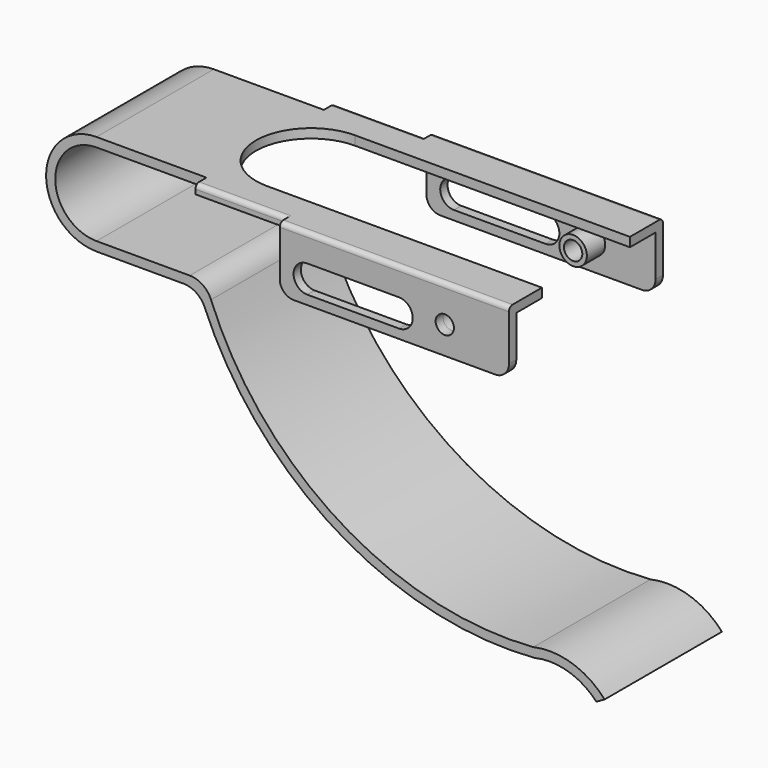
from build123d import *

# Parameters (mm, degrees)
F1_DEPTH  = 16
F2_W      = 70
F2_H      = 3
F3_DEPTH  = 2
F4_W      = 50
F4_H      = 14
F5_DEPTH  = 2
F6_R      = 1
F9_DEPTH  = 2
F11_DEPTH = 42.001
F13_D     = 4
F14_R     = 3
F14_R_2   = 2
F15_DEPTH = 5
F16_R     = 3


# Not quite as in the source:
# - a pattern or mirror of a feature is missing from the dataset's text; its kind, count and spacing are read off the source's solid


with BuildPart() as f1:
    # F0 (on Front) → F1 (new body)
    with BuildSketch(Plane.XZ):
        with BuildLine():
            ThreePointArc((0, -9), (-9, 0), (0, 9))
            Line((0, 9), (94, 9))
            Line((94, 9), (94, 11))
            Line((94, 11), (0, 11))
            ThreePointArc((0, 11), (-11, 0), (0, -11))
            Line((0, -11), (19, -11))
            ThreePointArc((19, -11), (21.7681124643, -11.8361612201), (23.6103896104, -14.064978646))
            ThreePointArc((23.6103896104, -14.064978646), (52.5045279084, -47.666837229), (95.6038093767, -57.9822657286))
            ThreePointArc((95.6038093767, -57.9822657286), (102.8775016632, -58.177663117), (109.0707194958, -61.9971961375))
            Line((109.0707194958, -61.9971961375), (110.8678187413, -61))
            ThreePointArc((110.8678187413, -61), (103.7692922231, -56.3602117831), (95.2965735981, -56))
            ThreePointArc((95.2965735981, -56), (52.955209083, -45.5949761441), (24.9861322889, -12.1467114099))
            ThreePointArc((24.9861322889, -12.1467114099), (23.1470623984, -9.8607704249), (20.3422845953, -9))
            Line((20.3422845953, -9), (0, -9))
        make_face()
    extrude(amount=F1_DEPTH)

    # F2 (on face) → F3 (join)
    with BuildSketch(Plane.XY.offset(11)):
        with Locations((59, -17.5)):
            Rectangle(F2_W, F2_H)
    extrude(amount=-F3_DEPTH)

    # F4 (on face) → F5 (join)
    with BuildSketch(Plane.XZ.offset(19)):
        with Locations((69, 4)):
            Rectangle(F4_W, F4_H)
    extrude(amount=F5_DEPTH)

    # F6
    f6_edges = [f1.edges().sort_by_distance(p)[0] for p in [
        (69, -21, 11),
        (34, -19, 11),
    ]]
    fillet(f6_edges, radius=F6_R)

    # F7: F1 across plane


with BuildPart() as f1_1:
    add(f1.part)
    add(f1.part.mirror(Plane.XZ))

    # F8 (on face) → F9 (cut)
    with BuildSketch(Plane.XY.offset(11)):
        with BuildLine():
            Line((94, 12), (34, 12))
            ThreePointArc((34, 12), (22, 0), (34, -12))
            Line((34, -12), (94, -12))
            Line((94, -12), (94, 12))
        make_face()
    extrude(amount=-F9_DEPTH, mode=Mode.SUBTRACT)

    # F10 (on face) → F11 (cut, through all)
    with BuildSketch(Plane.XZ.offset(21)):
        with BuildLine():
            ThreePointArc((50, 5), (47, 2), (50, -1))
            Line((50, -1), (70, -1))
            ThreePointArc((70, -1), (73, 2), (70, 5))
            Line((70, 5), (50, 5))
        make_face()
    extrude(amount=-F11_DEPTH, mode=Mode.SUBTRACT)

    # F13 (through all)
    with Locations(Plane.XZ.offset(21)):
        with Locations((80, 3)):
            Hole(F13_D / 2)

    # F14 (on face) → F15 (join)
    with BuildSketch(Plane(origin=(0, -19, 0), x_dir=(-1, 0, 0), z_dir=(0, 1, 0))):
        with Locations((-80, 3)):
            Circle(F14_R)
        with Locations((-80, 3)):
            Circle(F14_R_2, mode=Mode.SUBTRACT)
    f15 = extrude(amount=F15_DEPTH)

    # F15_copies: F15 across plane
    add(f15.mirror(Plane.ZX))

    # F16
    f16_edges = [f1_1.edges().sort_by_distance(p)[0] for p in [
        (44, -20, -3),
        (94, -20, -3),
        (94, 20, -3),
        (44, 20, -3),
    ]]
    fillet(f16_edges, radius=F16_R)


solid = f1_1.part
